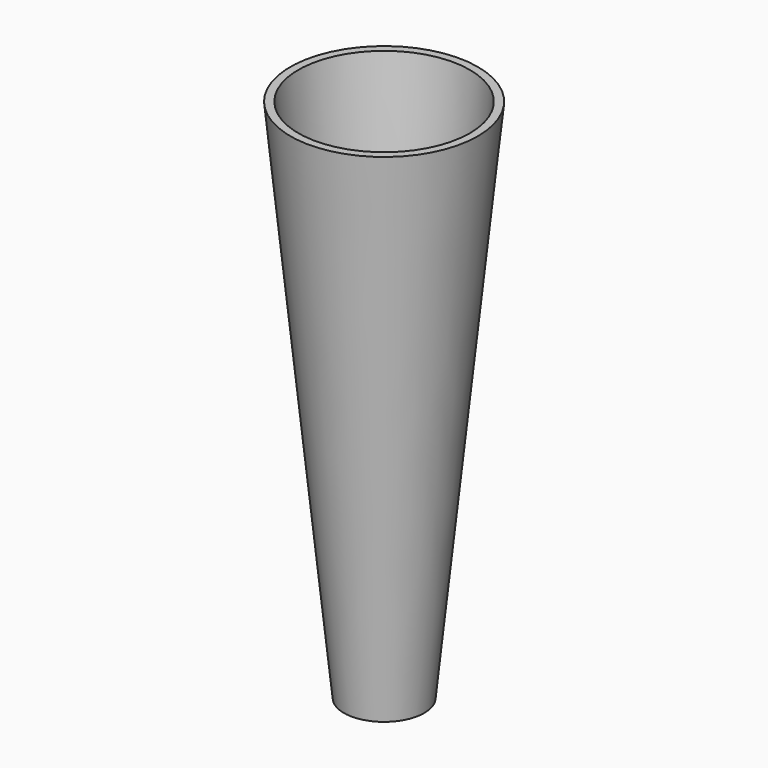
from build123d import *

# Parameters (mm, degrees)
F0_R = 9.525
F2_R = 22.225
F5_R = 7.62
F4_R = 20.32


with BuildPart() as f3:
    # F0 (on Top) → F3 section 0
    with BuildSketch(Plane.XY):
        Circle(F0_R)
    # F2 (on offset) → F3 section 1
    with BuildSketch(Plane.XY.offset(124.46)):
        Circle(F2_R)
    loft()

    # F5 (on face) → F6 section 0
    with BuildSketch(Plane(origin=(0, 0, 0), x_dir=(1, 0, 0), z_dir=(0, 0, -1))):
        Circle(F5_R)
    # F4 (on face) → F6 section 1
    with BuildSketch(Plane.XY.offset(124.46)):
        Circle(F4_R)
    loft(mode=Mode.SUBTRACT)


solid = f3.part
